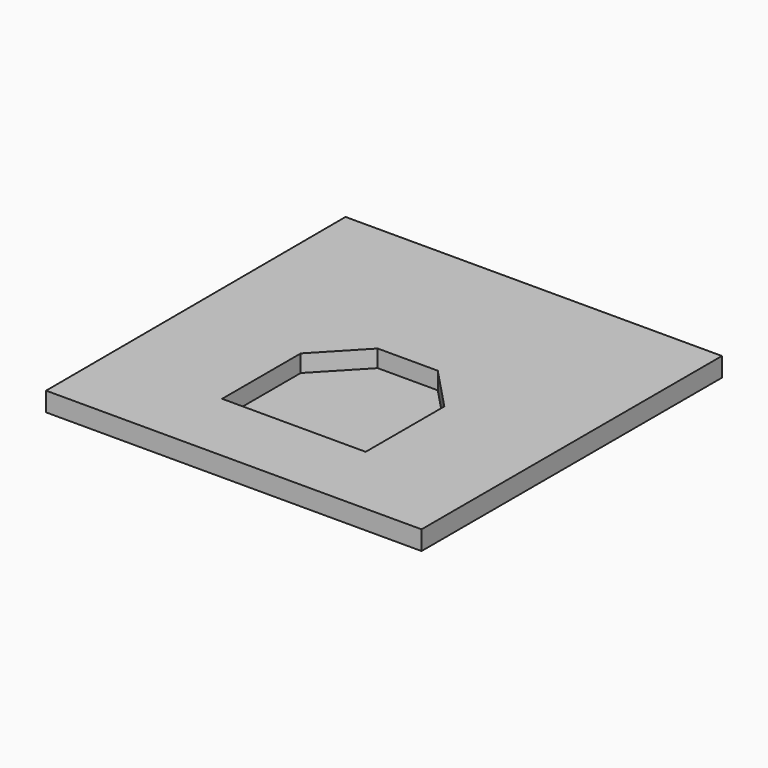
from build123d import *

# Parameters (mm, degrees)
F1_DEPTH = 230
F2_DEPTH = 25


# Not quite as in the source:
# - a feature names something its author has since deleted; it is built from what else it names


with BuildPart() as f1:
    # F0 (on Top) → F1 (new body)
    with BuildSketch(Plane.XY):
        Polygon((-2512.5771939687, 3487.8331422806), (-2500, -1512.1668577194), (2500, -1512.1668577194), (2500, 3487.8331422806), align=None)
        Polygon((-956, 796.8331971962), (-400, 1382.8331971962), (0, 1382.8331971962), (400, 1382.8331971962), (956, 796.8331971962), (956, -512.1668028038), (-956, -512.1668028038), align=None, mode=Mode.SUBTRACT)
    extrude(amount=F1_DEPTH)

    # F0 (on Top) → F2 (join)
    with BuildSketch(Plane.XY):
        Polygon((-2512.5771939687, 3487.8331422806), (-2500, -1512.1668577194), (2500, -1512.1668577194), (2500, 3487.8331422806), align=None)
        Polygon((-956, 796.8331971962), (-400, 1382.8331971962), (0, 1382.8331971962), (400, 1382.8331971962), (956, 796.8331971962), (956, -512.1668028038), (-956, -512.1668028038), align=None, mode=Mode.SUBTRACT)
        Polygon((0, 1382.8331971962), (-400, 1382.8331971962), (-956, 796.8331971962), (-956, -512.1668028038), (956, -512.1668028038), (956, 796.8331971962), (400, 1382.8331971962), align=None)
    extrude(amount=-F2_DEPTH)


solid = f1.part
